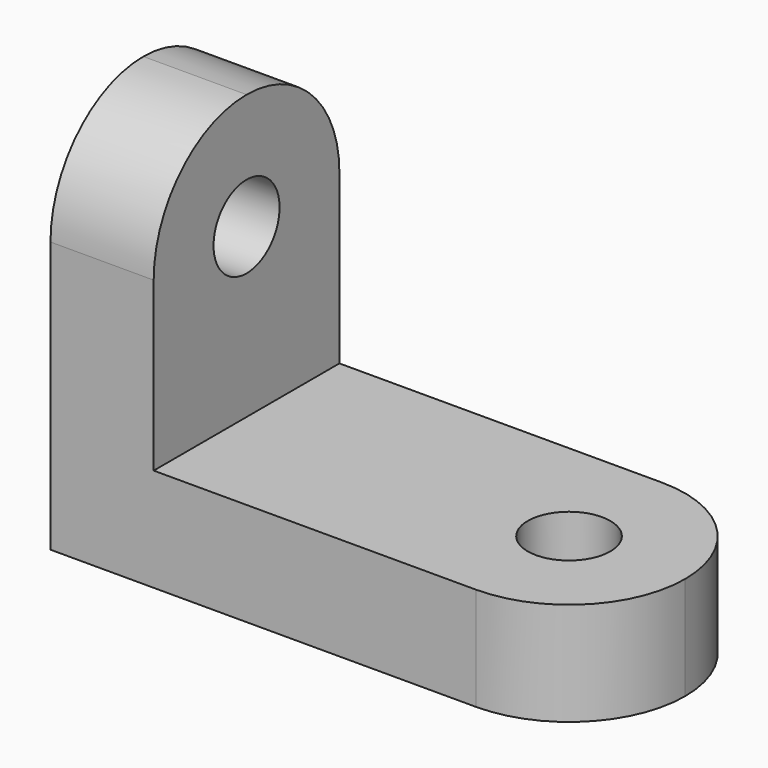
from build123d import *

# Parameters (mm, degrees)
F1_DEPTH = 9
F2_R     = 1.6
F3_DEPTH = 25
F4_R     = 1.6
F5_DEPTH = 25
F6_R     = 4.49999
F7_ANGLE = 90


# Not quite as in the source:
# - a fillet or chamfer is up to 0.001 mm smaller than in the source, because OpenCascade refuses the exact size


with BuildPart() as f1:
    # F0 (on Front) → F1 (new body)
    with BuildSketch(Plane.XZ):
        Polygon((-15, 4), (-15, 0), (0, 0), (0, 21), (-4, 21), (-4, 4), align=None)
    extrude(amount=F1_DEPTH)

    # F2 (on face) → F3 (cut)
    with BuildSketch(Plane.XY.offset(4)):
        with Locations((-10.5, -4.5)):
            Circle(F2_R)
    extrude(amount=-F3_DEPTH, mode=Mode.SUBTRACT)

    # F4 (on face) → F5 (cut)
    with BuildSketch(Plane(origin=(-4, 0, 0), x_dir=(0, -1, 0), z_dir=(-1, 0, 0))):
        with Locations((4.5, 16.5)):
            Circle(F4_R)
    extrude(amount=-F5_DEPTH, mode=Mode.SUBTRACT)

    # F6 (radius 4.5 in the source; OpenCascade refuses exactly that, so slightly less here)
    f6_edges = [f1.edges().sort_by_distance(p)[0] for p in [
        (-2, -9, 21),
        (-2, 0, 21),
        (-15, 0, 2),
        (-15, -9, 2),
    ]]
    fillet(f6_edges, radius=F6_R)


with BuildPart() as f1_1:
    # F7: moved
    add(f1.part.rotate(Axis((0, -4.5, 0), (0, 1, 0)), F7_ANGLE))


solid = f1_1.part
